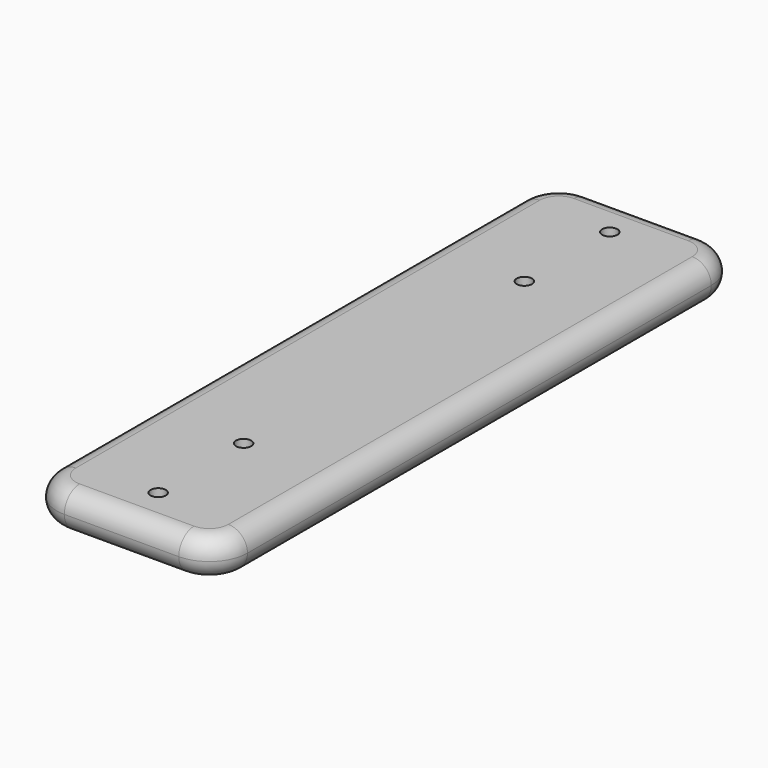
from build123d import *

# Parameters (mm, degrees)
F0_W     = 25
F0_H     = 43
F1_DEPTH = 5
F2_R     = 1
F3_DEPTH = 5.001
F4_R     = 5
F5_R     = 2.49999
F6_R     = 3
F7_DEPTH = 2


# Not quite as in the source:
# - a fillet or chamfer is up to 0.001 mm smaller than in the source, because OpenCascade refuses the exact size


with BuildPart() as f1:
    # F0 (on Top) → F1 (new body)
    with BuildSketch(Plane.XY):
        with Locations((0, 21.5)):
            Rectangle(F0_W, F0_H)
    extrude(amount=-F1_DEPTH)

    # F2 (on face) → F3 (cut, through all)
    with BuildSketch(Plane.XY):
        with Locations((0, 37)):
            Circle(F2_R)
        with Locations((0, 23)):
            Circle(F2_R)
    extrude(amount=-F3_DEPTH, mode=Mode.SUBTRACT)

    # F4
    f4_edges = [f1.edges().sort_by_distance(p)[0] for p in [
        (-12.5, 43, -2.5),
        (12.5, 43, -2.5),
    ]]
    fillet(f4_edges, radius=F4_R)

    # F5 (radius 2.5 in the source; OpenCascade refuses exactly that, so slightly less here)
    f5_edges = [f1.edges().sort_by_distance(p)[0] for p in [
        (-12.5, 19, 0),
        (-12.5, 19, -5),
    ]]
    fillet(f5_edges, radius=F5_R)

    # F6 (on face) → F7 (cut)
    with BuildSketch(Plane(origin=(0, 0, -5), x_dir=(1, 0, 0), z_dir=(0, 0, -1))):
        with Locations((0, -37)):
            Circle(F6_R)
        with Locations((0, -23)):
            Circle(F6_R)
    extrude(amount=-F7_DEPTH, mode=Mode.SUBTRACT)

    # F8: F1 across plane


with BuildPart() as f1_1:
    add(f1.part)
    add(f1.part.mirror(Plane.XZ))


solid = f1_1.part
